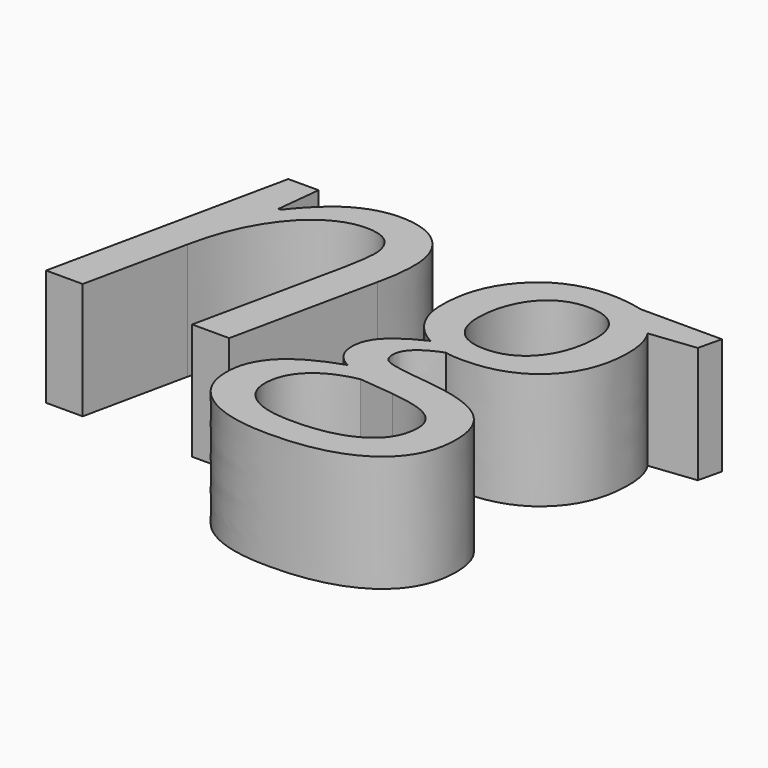
from build123d import *

# Parameters (mm, degrees)
F0_TEXT_SIZE = 38.3211726633
F1_DEPTH     = 10


# Not quite as in the source:
# - Text() gives the source's letters only with a copy of the font that has no kerning and outlines rounded to 1/6400 em; it was checked with that copy


with BuildPart() as f1:
    # F0 (on Top) → F1 (new body)
    with BuildSketch(Plane.XY):
        with Locations((-57.3380477726, 11.3526461646)):
            Text('ng', F0_TEXT_SIZE, font='Open Sans', font_style=FontStyle.ITALIC, text_align=(TextAlign.LEFT, TextAlign.BOTTOM))
    extrude(amount=F1_DEPTH)


solid = f1.part
